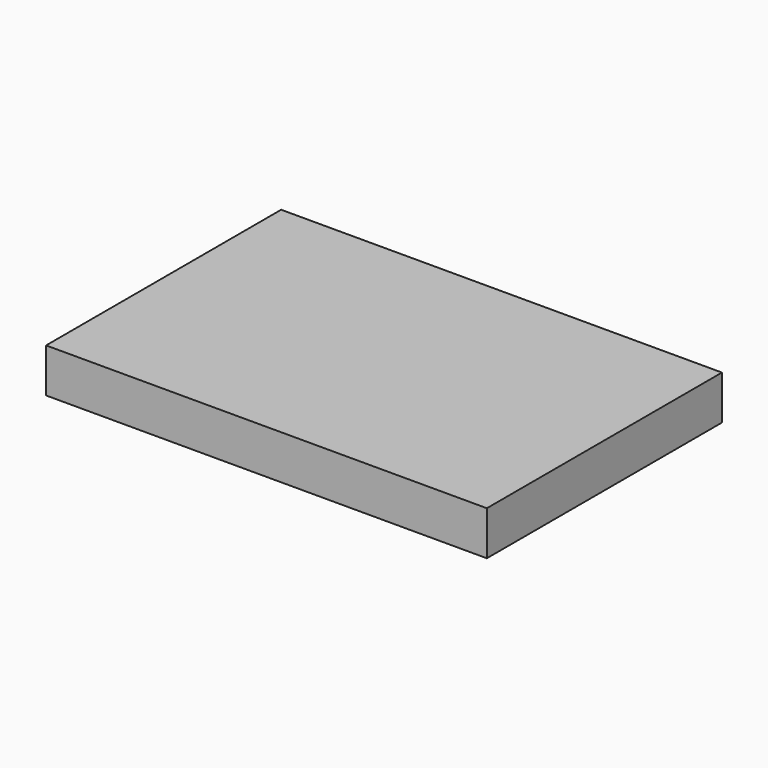
from build123d import *

# Parameters (mm, degrees)
F0_W     = 60
F0_H     = 40
F1_DEPTH = 3
F2_W     = 56
F2_H     = 36
F3_DEPTH = 3


with BuildPart() as f1:
    # F0 (on Top) → F1 (new body, symmetric)
    with BuildSketch(Plane.XY):
        Rectangle(F0_W, F0_H)
    extrude(amount=F1_DEPTH, both=True)

    # F2 (on face) → F3 (cut)
    with BuildSketch(Plane(origin=(0, 0, -3), x_dir=(1, 0, 0), z_dir=(0, 0, -1))):
        Rectangle(F2_W, F2_H)
    extrude(amount=-F3_DEPTH, mode=Mode.SUBTRACT)


solid = f1.part
